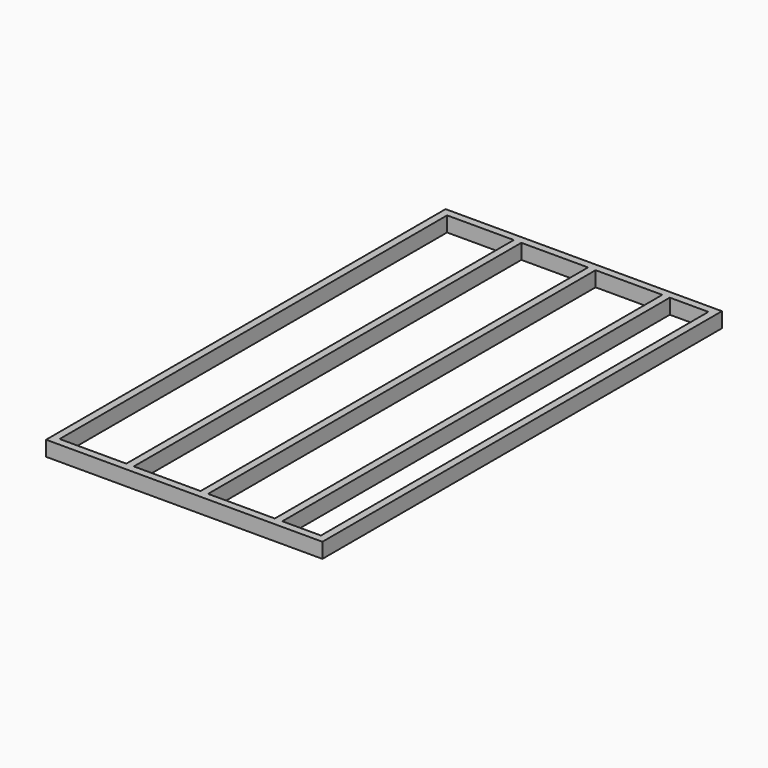
from build123d import *

# Parameters (mm, degrees)
F0_W     = 1512.7224
F0_H     = 2733.7512
F0_W_2   = 41.148
F0_H_2   = 2651.4552
F1_DEPTH = 82.55


# Not quite as in the source:
# - a feature names something its author has since deleted; it is built from what else it names


with BuildPart() as f1:
    # F0 (on Top) → F1 (new body)
    with BuildSketch(Plane.XY):
        Rectangle(F0_W, F0_H)
        Polygon((715.2132, 1325.7276), (715.2132, -1325.7276), (503.9868, -1325.7276), (462.8388, -1325.7276), (97.5868, -1325.7276), (56.4388, -1325.7276), (-308.8132, -1325.7276), (-349.9612, -1325.7276), (-715.2132, -1325.7276), (-715.2132, 1325.7276), (-349.9612, 1325.7276), (-308.8132, 1325.7276), (56.4388, 1325.7276), (97.5868, 1325.7276), (462.8388, 1325.7276), (503.9868, 1325.7276), align=None, mode=Mode.SUBTRACT)
        with Locations((483.4128, 0)):
            Rectangle(F0_W_2, F0_H_2)
        with Locations((77.0128, 0)):
            Rectangle(F0_W_2, F0_H_2)
        with Locations((-329.3872, 0)):
            Rectangle(F0_W_2, F0_H_2)
    extrude(amount=F1_DEPTH)


solid = f1.part
